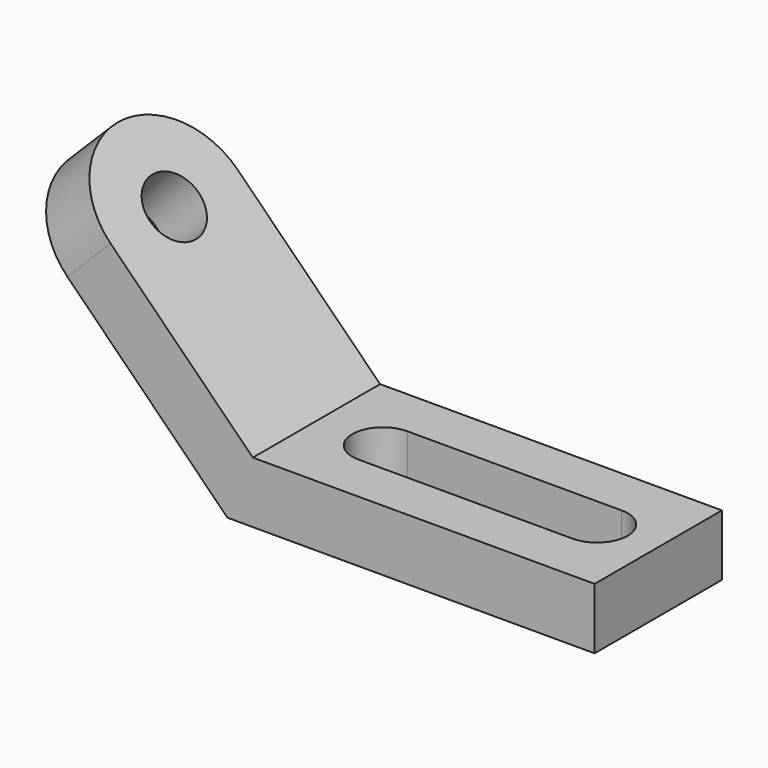
from build123d import *

# Parameters (mm, degrees)
F1_DEPTH = 52
F2_R     = 10
F3_DEPTH = 20
F5_DEPTH = 20
F6_R     = 25.99999


# Not quite as in the source:
# - a fillet or chamfer is up to 0.001 mm smaller than in the source, because OpenCascade refuses the exact size


with BuildPart() as f1:
    # F0 (on Front) → F1 (new body)
    with BuildSketch(Plane.XZ):
        Polygon((60.2885049582, -11.8481526151), (60.2885049582, 8.1518473849), (-51.4272237944, 8.1518473849), (-116.2800375368, 73.0046611273), (-130.4221731605, 58.8625255035), (-59.7114950418, -11.8481526151), align=None)
    extrude(amount=F1_DEPTH)

    # F2 (on face) → F3 (cut)
    with BuildSketch(Plane(origin=(-21.6376882048, 0, -21.6376882048), x_dir=(0.7071067812, 0, -0.7071067812), z_dir=(0.7071067812, 0, 0.7071067812))):
        with Locations((-107.8444940002, -26)):
            Circle(F2_R)
    extrude(amount=-F3_DEPTH, mode=Mode.SUBTRACT)

    # F4 (on face) → F5 (cut)
    with BuildSketch(Plane.XY.offset(8.1518473849)):
        with BuildLine():
            ThreePointArc((40.2885049582, -36), (47.35957277, -33.0710678119), (50.2885049582, -26))
            ThreePointArc((50.2885049582, -26), (47.35957277, -18.9289321881), (40.2885049582, -16))
            ThreePointArc((40.2885049582, -16), (30.2885049582, -26), (40.2885049582, -36))
        make_face()
        with BuildLine():
            ThreePointArc((40.2885049582, -36), (30.2885049582, -26), (40.2885049582, -16))
            Line((40.2885049582, -16), (-29.7114950418, -16))
            ThreePointArc((-29.7114950418, -16), (-22.64042723, -18.9289321881), (-19.7114950418, -26))
            ThreePointArc((-19.7114950418, -26), (-22.64042723, -33.0710678119), (-29.7114950418, -36))
            Line((-29.7114950418, -36), (40.2885049582, -36))
        make_face()
        with BuildLine():
            ThreePointArc((-19.7114950418, -26), (-22.64042723, -18.9289321881), (-29.7114950418, -16))
            ThreePointArc((-29.7114950418, -16), (-39.7114950418, -26), (-29.7114950418, -36))
            ThreePointArc((-29.7114950418, -36), (-22.64042723, -33.0710678119), (-19.7114950418, -26))
        make_face()
    extrude(amount=-F5_DEPTH, mode=Mode.SUBTRACT)

    # F6 (radius 26 in the source; OpenCascade refuses exactly that, so slightly less here)
    f6_edges = [f1.edges().sort_by_distance(p)[0] for p in [
        (-123.351105, -52, 65.933593),
        (-123.351105, 0, 65.933593),
    ]]
    fillet(f6_edges, radius=F6_R)


solid = f1.part
